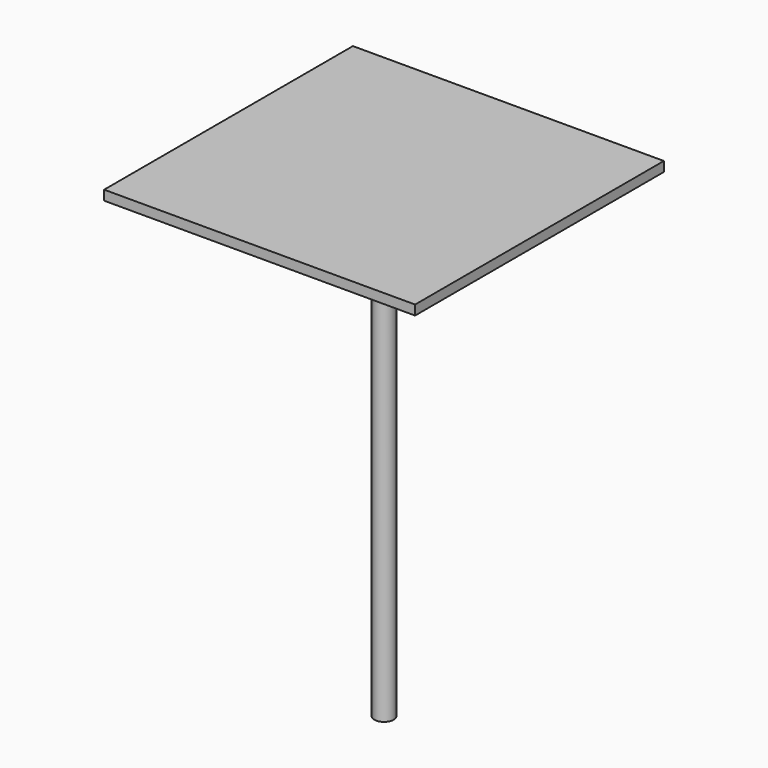
from build123d import *

# Parameters (mm, degrees)
F0_R     = 25
F1_DEPTH = 1000
F2_R     = 75
F2_R_2   = 25
F3_DEPTH = 200
F4_W     = 800
F4_H     = 800
F5_DEPTH = 25


with BuildPart() as f1:
    # F0 (on Top) → F1 (new body)
    with BuildSketch(Plane.XY):
        Circle(F0_R)
    extrude(amount=F1_DEPTH)

    # F2 (on face) → F3 (join)
    with BuildSketch(Plane.XY.offset(1000)):
        Circle(F2_R)
        Circle(F2_R_2, mode=Mode.SUBTRACT)
        Circle(F2_R_2)
    extrude(amount=F3_DEPTH)

    # F4 (on face) → F5 (join)
    with BuildSketch(Plane.XY.offset(1200)):
        Rectangle(F4_W, F4_H)
    extrude(amount=F5_DEPTH)


solid = f1.part
